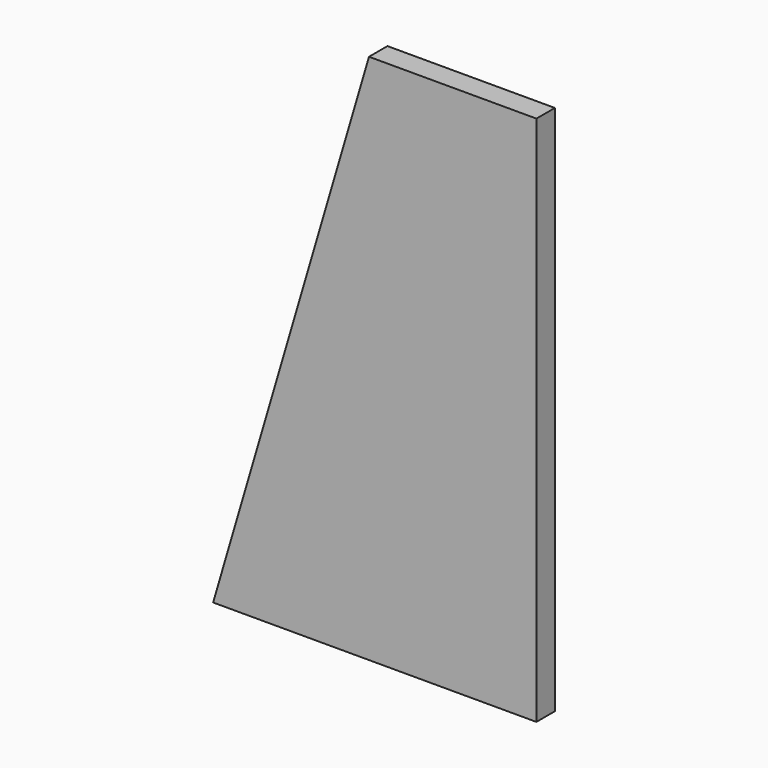
from build123d import *

# Parameters (mm, degrees)
F0_W     = 177.8
F0_H     = 292.1
F1_DEPTH = 12.7
F2_SIZE2 = 85.72499
F2_SIZE  = 292.09999


# Not quite as in the source:
# - a fillet or chamfer is up to 0.001 mm smaller than in the source, because OpenCascade refuses the exact size


with BuildPart() as f1:
    # F0 (on Front) → F1 (new body)
    with BuildSketch(Plane.XZ):
        Rectangle(F0_W, F0_H)
    extrude(amount=F1_DEPTH)

    # F2 (size 292.1 and 85.725 in the source; OpenCascade refuses exactly that, so slightly less here)
    f2_edges = [f1.edges().sort_by_distance(p)[0] for p in [
        (-88.9, -6.35, 146.05),
    ]]
    f2_side = f1.faces().sort_by_distance((-88.9, -6.35, 0))[0]
    chamfer(f2_edges, length=F2_SIZE, length2=F2_SIZE2, reference=f2_side)


solid = f1.part
